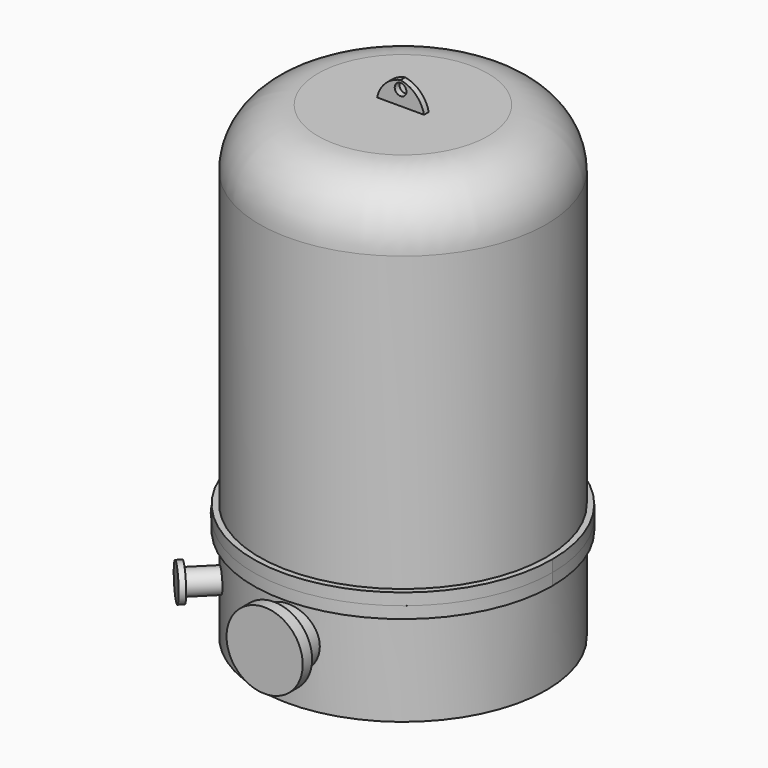
from build123d import *

# Parameters (mm, degrees)
F0_R           = 311.15
F0_R_2         = 298.45
F1_DEPTH       = 177.8
F2_R           = 323.85
F2_R_2         = 298.45
F3_DEPTH       = 25.4
F5_R           = 63.5
F6_DEPTH       = 44.45
F6_DEPTH_BACK  = 25.4
F7_R           = 82.55
F8_DEPTH       = 25.4
F10_R          = 25.4
F11_DEPTH      = 7.62
F11_DEPTH_BACK = 68.58
F12_R          = 38.1
F13_DEPTH      = 12.7
F14_COUNT      = 2
F14_ANGLE      = 45
F15_COUNT      = 2
F15_ANGLE      = 45
F16_R          = 323.85
F16_R_2        = 298.45
F17_DEPTH      = 25.4
F18_R          = 311.15
F18_R_2        = 298.45
F19_DEPTH      = 685.8
F20_R          = 311.15
F21_DEPTH      = 76.2
F22_R          = 109.5375
F23_DEPTH      = 63.5
F25_W          = 101.6
F25_H          = 12.7
F26_DEPTH      = 50.8
F28_T1_DEPTH   = 323.7851973335
F29_R          = 127
F31_W          = 50.8
F31_H          = 25.4
F32_DEPTH      = 25.4
F33_W          = 50.8
F33_H          = 25.4
F34_DEPTH      = 25.4
F35_R          = 311.15
F36_DEPTH      = 25
F27_R          = 12.7
F37_DEPTH      = 25.4
F37_DEPTH_BACK = 25.4
F38_R          = 127
F39_DEPTH      = 12.7
F24_R          = 12.5
F24_R_2        = 96.8375
F40_DEPTH      = 254
F40_DEPTH_BACK = 254
F41_R          = 3.175
F42_DEPTH      = 12.7
F43_W          = 25.4
F43_H          = 25.4
F44_DEPTH      = 152.4
F45_R          = 193.675
F46_DEPTH      = 12.7
F47_R          = 3.175
F48_DEPTH      = 12.446


# Not quite as in the source:
# - a fillet or chamfer that OpenCascade refuses, or shapes differently, is made with other operations: its cross-section is extruded or revolved along the edge and cut away or added


with BuildPart() as f1:
    # F0 (on Top) → F1 (new body)
    with BuildSketch(Plane.XY):
        Circle(F0_R)
        Circle(F0_R_2, mode=Mode.SUBTRACT)
    extrude(amount=F1_DEPTH)

    # F2 (on face) → F3 (join)
    with BuildSketch(Plane.XY.offset(177.8)):
        Circle(F2_R)
        Circle(F2_R_2, mode=Mode.SUBTRACT)
    extrude(amount=F3_DEPTH)

    # F5 (on offset) → F6 (join, two sides)
    with BuildSketch(Plane.XZ.offset(304.8)) as f6_sk:
        with Locations((0, 101.6)):
            Circle(F5_R)
    extrude(amount=F6_DEPTH)
    extrude(f6_sk.sketch, amount=-F6_DEPTH_BACK)

    # F7 (on face) → F8 (join)
    with BuildSketch(Plane.XZ.offset(349.25)):
        with Locations((0, 101.6)):
            Circle(F7_R)
    extrude(amount=F8_DEPTH)

    # F31 (on offset) → F32 (join)
    with BuildSketch(Plane.YZ.offset(-342.9)):
        with Locations((9.0822450161, 190.5)):
            Rectangle(F31_W, F31_H)
    extrude(amount=F32_DEPTH)



with BuildPart() as f11:
    # F10 (on offset) → F11 (new body, two sides)
    with BuildSketch(Plane.YZ.offset(-304.8)) as f11_sk:
        with Locations((0, 101.6)):
            Circle(F10_R)
    extrude(amount=F11_DEPTH)
    extrude(f11_sk.sketch, amount=-F11_DEPTH_BACK)

    # F12 (on face) → F13 (join)
    with BuildSketch(Plane(origin=(-373.38, 0, 0), x_dir=(0, -1, 0), z_dir=(-1, 0, 0))):
        with Locations((0, 101.6)):
            Circle(F12_R)
    extrude(amount=F13_DEPTH)


with BuildPart() as f14_1:
    # F14: instance of F11
    add(f11.part.rotate(Axis((0, 0, 0), (0, 0, -1)), 1 * F14_ANGLE / (F14_COUNT - 1)))


with BuildPart() as f15_1:
    # F15: instance of F11
    add(f11.part.rotate(Axis((0, 0, 0), (0, 0, 1)), 1 * F15_ANGLE / (F15_COUNT - 1)))


with BuildPart() as f17:
    # F16 (on face) → F17 (new body)
    with BuildSketch(Plane.XY.offset(203.2)):
        Circle(F16_R)
        Circle(F16_R_2, mode=Mode.SUBTRACT)
    extrude(amount=F17_DEPTH)

    # F18 (on face) → F19 (join)
    with BuildSketch(Plane.XY.offset(228.6)):
        Circle(F18_R)
        Circle(F18_R_2, mode=Mode.SUBTRACT)
    extrude(amount=F19_DEPTH)

    # F20 (on face) → F21 (join)
    with BuildSketch(Plane.XY.offset(914.4)):
        Circle(F20_R)
    extrude(amount=F21_DEPTH)

    # F25 (on face) → F26 (join)
    with BuildSketch(Plane.XY.offset(990.6)):
        Rectangle(F25_W, F25_H)
    extrude(amount=F26_DEPTH)

    # F28: fillet of radius 63.5 on 2 edges, made by hand

    # F28_s2 → F28_t1 (cut)
    with BuildSketch(Plane.XZ.offset(-161.8925986667)):
        with BuildLine():
            ThreePointArc((50.8, 990.6), (28.7438868174, 1027.0868884968), (-11.4170394667, 1041.4))
            Line((-11.4170394667, 1041.4), (50.8, 1041.4))
            Line((50.8, 1041.4), (50.8, 990.6))
        make_face()
        with BuildLine():
            ThreePointArc((-50.8, 990.6), (-28.7438868174, 1027.0868884968), (11.4170394667, 1041.4))
            Line((11.4170394667, 1041.4), (-50.8, 1041.4))
            Line((-50.8, 1041.4), (-50.8, 990.6))
        make_face()
    extrude(amount=F28_T1_DEPTH, mode=Mode.SUBTRACT)

    # F29
    f29_edges = [f17.edges().sort_by_distance(p)[0] for p in [
        (-311.15, 0, 990.6),
    ]]
    fillet(f29_edges, radius=F29_R)

    # F33 (on offset) → F34 (join)
    with BuildSketch(Plane.YZ.offset(-342.9)):
        with Locations((9.6526147002, 215.9)):
            Rectangle(F33_W, F33_H)
    extrude(amount=F34_DEPTH)

    # F27 (on face) → F37 (cut, two sides)
    with BuildSketch(Plane.XZ.offset(6.35)) as f37_sk:
        with Locations((0, 1022.35)):
            Circle(F27_R)
    extrude(amount=-F37_DEPTH, mode=Mode.SUBTRACT)
    extrude(f37_sk.sketch, amount=F37_DEPTH_BACK, mode=Mode.SUBTRACT)


with BuildPart() as f23:
    # F22 (on face) → F23 (new body)
    with BuildSketch(Plane(origin=(0, 0, 0), x_dir=(1, 0, 0), z_dir=(0, 0, -1))):
        Circle(F22_R)
    extrude(amount=F23_DEPTH)


with BuildPart() as f1_1:
    add(f1.part)

    add(f23.part)  # F36 merges F23
    # F35 (on face) → F36 (join)
    with BuildSketch(Plane(origin=(0, 0, 0), x_dir=(1, 0, 0), z_dir=(0, 0, -1))):
        Circle(F35_R)
    extrude(amount=F36_DEPTH)

    # F38 (on face) → F39 (join)
    with BuildSketch(Plane(origin=(0, 0, -63.5), x_dir=(1, 0, 0), z_dir=(0, 0, -1))):
        Circle(F38_R)
    extrude(amount=F39_DEPTH)

    # F24 (on face) → F40 (cut, two sides)
    with BuildSketch(Plane(origin=(0, 0, 0), x_dir=(1, 0, 0), z_dir=(0, 0, -1))) as f40_sk:
        with Locations((50.7179116105, -141.8161436442)):
            Circle(F24_R)
        with Locations((-64.4161776252, -136.1421360799)):
            Circle(F24_R)
        with Locations((-141.8161436442, -50.7179116105)):
            Circle(F24_R)
        with Locations((-136.1421360799, 64.4161776252)):
            Circle(F24_R)
        with Locations((-50.7179116105, 141.8161436442)):
            Circle(F24_R)
        Circle(F24_R_2)
    extrude(amount=-F40_DEPTH, mode=Mode.SUBTRACT)
    extrude(f40_sk.sketch, amount=F40_DEPTH_BACK, mode=Mode.SUBTRACT)

    # F41 (on face) → F42 (cut)
    with BuildSketch(Plane.XY):
        with Locations((-92.075, 92.075)):
            Circle(F41_R)
        with Locations((92.075, 92.075)):
            Circle(F41_R)
        with Locations((92.075, -92.075)):
            Circle(F41_R)
        with Locations((-92.075, -92.075)):
            Circle(F41_R)
    extrude(amount=-F42_DEPTH, mode=Mode.SUBTRACT)


with BuildPart() as f44:
    # F43 (on face) → F44 (new body)
    with BuildSketch(Plane.XY):
        with Locations((-92.075, 92.075)):
            Rectangle(F43_W, F43_H)
    extrude(amount=F44_DEPTH)



with BuildPart() as f44b:
    # F43 (on face) → F44, piece 2 (new body)
    with BuildSketch(Plane.XY):
        with Locations((92.075, 92.075)):
            Rectangle(F43_W, F43_H)
    extrude(amount=F44_DEPTH)


with BuildPart() as f44c:
    # F43 (on face) → F44, piece 3 (new body)
    with BuildSketch(Plane.XY):
        with Locations((92.075, -92.075)):
            Rectangle(F43_W, F43_H)
    extrude(amount=F44_DEPTH)


with BuildPart() as f44d:
    # F43 (on face) → F44, piece 4 (new body)
    with BuildSketch(Plane.XY):
        with Locations((-92.075, -92.075)):
            Rectangle(F43_W, F43_H)
    extrude(amount=F44_DEPTH)


with BuildPart() as f44_1:
    add(f44.part)

    add(f44b.part)  # F46 merges F44b

    add(f44c.part)  # F46 merges F44c

    add(f44d.part)  # F46 merges F44d
    # F45 (on face) → F46 (join)
    with BuildSketch(Plane.XY.offset(152.4)):
        Circle(F45_R)
    extrude(amount=F46_DEPTH)

    # F47 (on face) → F48 (cut)
    with BuildSketch(Plane.XY.offset(165.1)):
        Circle(F47_R)
        with Locations((0, 25.4)):
            Circle(F47_R)
        with Locations((0, 50.8)):
            Circle(F47_R)
        with Locations((0, 76.2)):
            Circle(F47_R)
        with Locations((0, 101.6)):
            Circle(F47_R)
        with Locations((0, 127)):
            Circle(F47_R)
        with Locations((0, 152.4)):
            Circle(F47_R)
        with Locations((25.4, 0)):
            Circle(F47_R)
        with Locations((25.4, 25.4)):
            Circle(F47_R)
        with Locations((25.4, 50.8)):
            Circle(F47_R)
        with Locations((25.4, 76.2)):
            Circle(F47_R)
        with Locations((25.4, 101.6)):
            Circle(F47_R)
        with Locations((25.4, 127)):
            Circle(F47_R)
        with Locations((25.4, 152.4)):
            Circle(F47_R)
        with Locations((50.8, 0)):
            Circle(F47_R)
        with Locations((50.8, 25.4)):
            Circle(F47_R)
        with Locations((50.8, 50.8)):
            Circle(F47_R)
        with Locations((50.8, 76.2)):
            Circle(F47_R)
        with Locations((50.8, 101.6)):
            Circle(F47_R)
        with Locations((50.8, 127)):
            Circle(F47_R)
        with Locations((50.8, 152.4)):
            Circle(F47_R)
        with Locations((76.2, 0)):
            Circle(F47_R)
        with Locations((76.2, 25.4)):
            Circle(F47_R)
        with Locations((76.2, 50.8)):
            Circle(F47_R)
        with Locations((76.2, 76.2)):
            Circle(F47_R)
        with Locations((76.2, 101.6)):
            Circle(F47_R)
        with Locations((76.2, 127)):
            Circle(F47_R)
        with Locations((76.2, 152.4)):
            Circle(F47_R)
        with Locations((101.6, 0)):
            Circle(F47_R)
        with Locations((101.6, 25.4)):
            Circle(F47_R)
        with Locations((101.6, 50.8)):
            Circle(F47_R)
        with Locations((101.6, 76.2)):
            Circle(F47_R)
        with Locations((101.6, 101.6)):
            Circle(F47_R)
        with Locations((101.6, 127)):
            Circle(F47_R)
        with Locations((101.6, 152.4)):
            Circle(F47_R)
        with Locations((127, 0)):
            Circle(F47_R)
        with Locations((127, 25.4)):
            Circle(F47_R)
        with Locations((127, 50.8)):
            Circle(F47_R)
        with Locations((127, 76.2)):
            Circle(F47_R)
        with Locations((127, 101.6)):
            Circle(F47_R)
        with Locations((127, 127)):
            Circle(F47_R)
        with Locations((127, 152.4)):
            Circle(F47_R)
        with Locations((152.4, 0)):
            Circle(F47_R)
        with Locations((152.4, 25.4)):
            Circle(F47_R)
        with Locations((152.4, 50.8)):
            Circle(F47_R)
        with Locations((152.4, 76.2)):
            Circle(F47_R)
        with Locations((152.4, 101.6)):
            Circle(F47_R)
        with Locations((152.4, 127)):
            Circle(F47_R)
        with Locations((152.4, 152.4)):
            Circle(F47_R)
        with Locations((-25.4, 0)):
            Circle(F47_R)
        with Locations((-25.4, 25.4)):
            Circle(F47_R)
        with Locations((-25.4, 50.8)):
            Circle(F47_R)
        with Locations((-25.4, 76.2)):
            Circle(F47_R)
        with Locations((-25.4, 101.6)):
            Circle(F47_R)
        with Locations((-25.4, 127)):
            Circle(F47_R)
        with Locations((-25.4, 152.4)):
            Circle(F47_R)
        with Locations((-50.8, 0)):
            Circle(F47_R)
        with Locations((-50.8, 25.4)):
            Circle(F47_R)
        with Locations((-50.8, 50.8)):
            Circle(F47_R)
        with Locations((-50.8, 76.2)):
            Circle(F47_R)
        with Locations((-50.8, 101.6)):
            Circle(F47_R)
        with Locations((-50.8, 127)):
            Circle(F47_R)
        with Locations((-50.8, 152.4)):
            Circle(F47_R)
        with Locations((-76.2, 0)):
            Circle(F47_R)
        with Locations((-76.2, 25.4)):
            Circle(F47_R)
        with Locations((-76.2, 50.8)):
            Circle(F47_R)
        with Locations((-76.2, 76.2)):
            Circle(F47_R)
        with Locations((-76.2, 101.6)):
            Circle(F47_R)
        with Locations((-76.2, 127)):
            Circle(F47_R)
        with Locations((-76.2, 152.4)):
            Circle(F47_R)
        with Locations((-101.6, 0)):
            Circle(F47_R)
        with Locations((-101.6, 25.4)):
            Circle(F47_R)
        with Locations((-101.6, 50.8)):
            Circle(F47_R)
        with Locations((-101.6, 76.2)):
            Circle(F47_R)
        with Locations((-101.6, 101.6)):
            Circle(F47_R)
        with Locations((-101.6, 127)):
            Circle(F47_R)
        with Locations((-101.6, 152.4)):
            Circle(F47_R)
        with Locations((-127, 0)):
            Circle(F47_R)
        with Locations((-127, 25.4)):
            Circle(F47_R)
        with Locations((-127, 50.8)):
            Circle(F47_R)
        with Locations((-127, 76.2)):
            Circle(F47_R)
        with Locations((-127, 101.6)):
            Circle(F47_R)
        with Locations((-127, 127)):
            Circle(F47_R)
        with Locations((-127, 152.4)):
            Circle(F47_R)
        with Locations((-152.4, 0)):
            Circle(F47_R)
        with Locations((-152.4, 25.4)):
            Circle(F47_R)
        with Locations((-152.4, 50.8)):
            Circle(F47_R)
        with Locations((-152.4, 76.2)):
            Circle(F47_R)
        with Locations((-152.4, 101.6)):
            Circle(F47_R)
        with Locations((-152.4, 127)):
            Circle(F47_R)
        with Locations((-152.4, 152.4)):
            Circle(F47_R)
        with Locations((0, -25.4)):
            Circle(F47_R)
        with Locations((0, -50.8)):
            Circle(F47_R)
        with Locations((0, -76.2)):
            Circle(F47_R)
        with Locations((0, -101.6)):
            Circle(F47_R)
        with Locations((0, -127)):
            Circle(F47_R)
        with Locations((0, -152.4)):
            Circle(F47_R)
        with Locations((25.4, -25.4)):
            Circle(F47_R)
        with Locations((25.4, -50.8)):
            Circle(F47_R)
        with Locations((25.4, -76.2)):
            Circle(F47_R)
        with Locations((25.4, -101.6)):
            Circle(F47_R)
        with Locations((25.4, -127)):
            Circle(F47_R)
        with Locations((25.4, -152.4)):
            Circle(F47_R)
        with Locations((50.8, -25.4)):
            Circle(F47_R)
        with Locations((50.8, -50.8)):
            Circle(F47_R)
        with Locations((50.8, -76.2)):
            Circle(F47_R)
        with Locations((50.8, -101.6)):
            Circle(F47_R)
        with Locations((50.8, -127)):
            Circle(F47_R)
        with Locations((50.8, -152.4)):
            Circle(F47_R)
        with Locations((76.2, -25.4)):
            Circle(F47_R)
        with Locations((76.2, -50.8)):
            Circle(F47_R)
        with Locations((76.2, -76.2)):
            Circle(F47_R)
        with Locations((76.2, -101.6)):
            Circle(F47_R)
        with Locations((76.2, -127)):
            Circle(F47_R)
        with Locations((76.2, -152.4)):
            Circle(F47_R)
        with Locations((101.6, -25.4)):
            Circle(F47_R)
        with Locations((101.6, -50.8)):
            Circle(F47_R)
        with Locations((101.6, -76.2)):
            Circle(F47_R)
        with Locations((101.6, -101.6)):
            Circle(F47_R)
        with Locations((101.6, -127)):
            Circle(F47_R)
        with Locations((101.6, -152.4)):
            Circle(F47_R)
        with Locations((127, -25.4)):
            Circle(F47_R)
        with Locations((127, -50.8)):
            Circle(F47_R)
        with Locations((127, -76.2)):
            Circle(F47_R)
        with Locations((127, -101.6)):
            Circle(F47_R)
        with Locations((127, -127)):
            Circle(F47_R)
        with Locations((127, -152.4)):
            Circle(F47_R)
        with Locations((152.4, -25.4)):
            Circle(F47_R)
        with Locations((152.4, -50.8)):
            Circle(F47_R)
        with Locations((152.4, -76.2)):
            Circle(F47_R)
        with Locations((152.4, -101.6)):
            Circle(F47_R)
        with Locations((152.4, -127)):
            Circle(F47_R)
        with Locations((152.4, -152.4)):
            Circle(F47_R)
        with Locations((-25.4, -25.4)):
            Circle(F47_R)
        with Locations((-25.4, -50.8)):
            Circle(F47_R)
        with Locations((-25.4, -76.2)):
            Circle(F47_R)
        with Locations((-25.4, -101.6)):
            Circle(F47_R)
        with Locations((-25.4, -127)):
            Circle(F47_R)
        with Locations((-25.4, -152.4)):
            Circle(F47_R)
        with Locations((-50.8, -25.4)):
            Circle(F47_R)
        with Locations((-50.8, -50.8)):
            Circle(F47_R)
        with Locations((-50.8, -76.2)):
            Circle(F47_R)
        with Locations((-50.8, -101.6)):
            Circle(F47_R)
        with Locations((-50.8, -127)):
            Circle(F47_R)
        with Locations((-50.8, -152.4)):
            Circle(F47_R)
        with Locations((-76.2, -25.4)):
            Circle(F47_R)
        with Locations((-76.2, -50.8)):
            Circle(F47_R)
        with Locations((-76.2, -76.2)):
            Circle(F47_R)
        with Locations((-76.2, -101.6)):
            Circle(F47_R)
        with Locations((-76.2, -127)):
            Circle(F47_R)
        with Locations((-76.2, -152.4)):
            Circle(F47_R)
        with Locations((-101.6, -25.4)):
            Circle(F47_R)
        with Locations((-101.6, -50.8)):
            Circle(F47_R)
        with Locations((-101.6, -76.2)):
            Circle(F47_R)
        with Locations((-101.6, -101.6)):
            Circle(F47_R)
        with Locations((-101.6, -127)):
            Circle(F47_R)
        with Locations((-101.6, -152.4)):
            Circle(F47_R)
        with Locations((-127, -25.4)):
            Circle(F47_R)
        with Locations((-127, -50.8)):
            Circle(F47_R)
        with Locations((-127, -76.2)):
            Circle(F47_R)
        with Locations((-127, -101.6)):
            Circle(F47_R)
        with Locations((-127, -127)):
            Circle(F47_R)
        with Locations((-127, -152.4)):
            Circle(F47_R)
        with Locations((-152.4, -25.4)):
            Circle(F47_R)
        with Locations((-152.4, -50.8)):
            Circle(F47_R)
        with Locations((-152.4, -76.2)):
            Circle(F47_R)
        with Locations((-152.4, -101.6)):
            Circle(F47_R)
        with Locations((-152.4, -127)):
            Circle(F47_R)
        with Locations((-152.4, -152.4)):
            Circle(F47_R)
    extrude(amount=-F48_DEPTH, mode=Mode.SUBTRACT)


solid = Compound([f11.part, f14_1.part, f15_1.part, f17.part, f1_1.part, f44_1.part])
